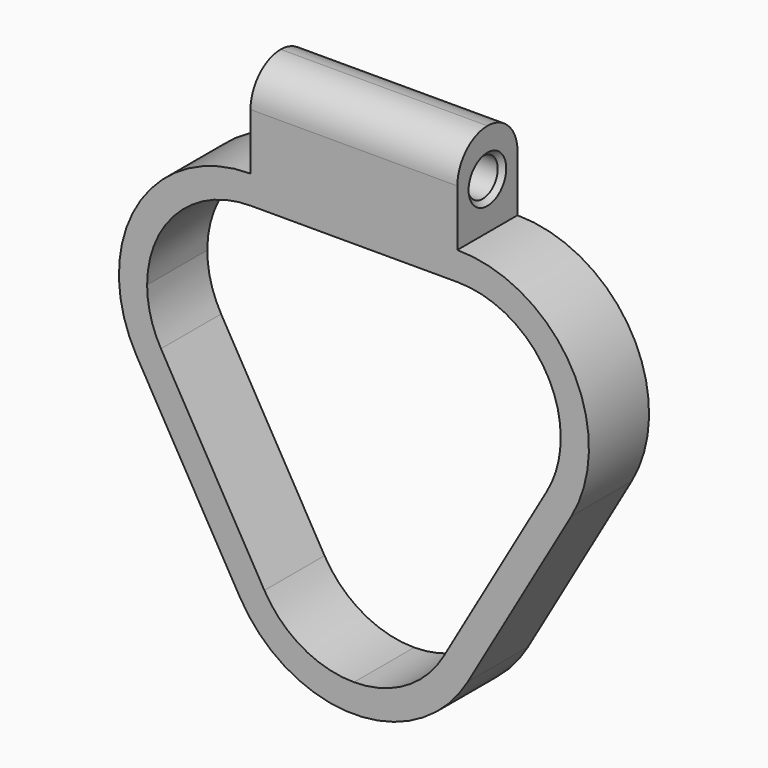
from build123d import *

# Parameters (mm, degrees)
F1_DEPTH       = 8
F2_DEPTH       = 10
F5_D           = 4
F5_DEPTH       = 12.7
F5_CSINK_D     = 5
F5_CSINK_ANGLE = 90
F5_TIP         = 1.2017212381
F6_D           = 4
F6_DEPTH       = 15
F6_CSINK_D     = 5
F6_CSINK_ANGLE = 90
F6_TIP         = 1.2017212381
F7_R           = 3.99999


# Not quite as in the source:
# - a fillet or chamfer is up to 0.001 mm smaller than in the source, because OpenCascade refuses the exact size


with BuildPart() as f1:
    # F0 (on Front) → F1 (new body)
    with BuildSketch(Plane.XZ):
        with BuildLine():
            ThreePointArc((0, 14), (-12.124355653, 7), (-12.124355653, -7))
            Line((-12.124355653, -7), (-1.124355653, -26.0525588833))
            ThreePointArc((-1.124355653, -26.0525588833), (11, -33.0525588833), (23.124355653, -26.0525588833))
            Line((23.124355653, -26.0525588833), (34.124355653, -7))
            ThreePointArc((34.124355653, -7), (34.124355653, 7), (22, 14))
            Line((22, 14), (0, 14))
        make_face()
        with BuildLine():
            ThreePointArc((-11, 0), (-7.7781745931, 7.7781745931), (0, 11))
            Line((0, 11), (11, 11))
            Line((11, 11), (22, 11))
            ThreePointArc((22, 11), (29.7781745931, 7.7781745931), (33, 0))
            ThreePointArc((33, 0), (32.6251840892, -2.8470094961), (31.5262794416, -5.5))
            Line((31.5262794416, -5.5), (20.5262794416, -24.5525588833))
            ThreePointArc((20.5262794416, -24.5525588833), (16.5, -28.5788383249), (11, -30.0525588833))
            ThreePointArc((11, -30.0525588833), (5.5, -28.5788383249), (1.4737205584, -24.5525588833))
            Line((1.4737205584, -24.5525588833), (-9.5262794416, -5.5))
            ThreePointArc((-9.5262794416, -5.5), (-10.6251840892, -2.8470094961), (-11, 0))
        make_face(mode=Mode.SUBTRACT)
    extrude(amount=F1_DEPTH)

    # F2 (add): a face of the model
    f2_faces = [f1.faces().sort_by_distance(p)[0] for p in [
        (11, -4, 14),
    ]]
    extrude(f2_faces, amount=F2_DEPTH)

    # F5
    with Locations(Plane.YZ.offset(22)):
        with Locations((-4, 19)):
            CounterSinkHole(F5_D / 2, F5_CSINK_D / 2, depth=F5_DEPTH, counter_sink_angle=F5_CSINK_ANGLE)
            with Locations((0, 0, -(F5_DEPTH + F5_TIP / 2))):  # 118° drill point
                Cone(0, F5_D / 2, F5_TIP, mode=Mode.SUBTRACT)

    # F6
    with Locations(Plane(origin=(0, 0, 0), x_dir=(0, -1, 0), z_dir=(-1, 0, 0))):
        with Locations((4, 19)):
            CounterSinkHole(F6_D / 2, F6_CSINK_D / 2, depth=F6_DEPTH, counter_sink_angle=F6_CSINK_ANGLE)
            with Locations((0, 0, -(F6_DEPTH + F6_TIP / 2))):  # 118° drill point
                Cone(0, F6_D / 2, F6_TIP, mode=Mode.SUBTRACT)

    # F7 (radius 4 in the source; OpenCascade refuses exactly that, so slightly less here)
    f7_edges = [f1.edges().sort_by_distance(p)[0] for p in [
        (11, 0, 24),
        (11, -8, 24),
    ]]
    fillet(f7_edges, radius=F7_R)


solid = f1.part
